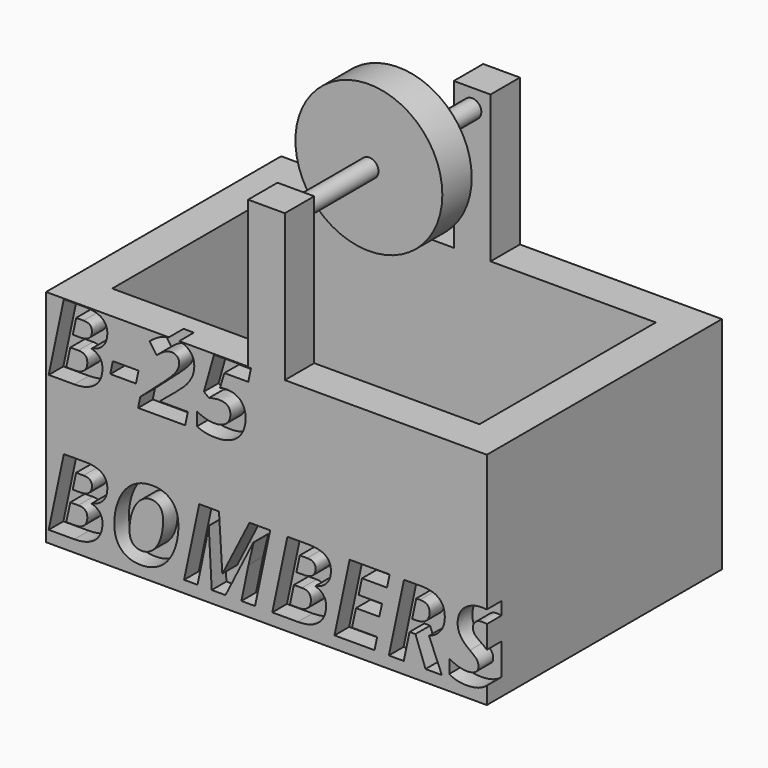
from build123d import *

# Parameters (mm, degrees)
F0_W          = 152.4
F0_H          = 76.2
F1_DEPTH      = 101.6
F2_W          = 127
F2_H          = 76.2
F3_DEPTH      = 63.5
F4_W          = 90.9743383527
F4_H          = 43.2646684349
F5_DEPTH      = 127
F6_W          = 12.7
F6_H          = 12.7
F7_DEPTH      = 50.8
F8_R          = 3.175
F9_DEPTH      = 101.6
F11_R         = 25.4
F12_DEPTH     = 6.35
F15_TEXT_SIZE = 34.6716756447
F16_DEPTH     = 6.35


# Not quite as in the source:
# - the program builds the solid bodies; features that only make, move or delete a surface that nothing else refers to are left out
# - Text() gives the source's letters only with a copy of the font that has no kerning and outlines rounded to 1/6400 em; it was checked with that copy


with BuildPart() as f1:
    # F0 (on Front) → F1 (new body)
    with BuildSketch(Plane.XZ):
        with Locations((-3.6829989403, -13.9763858854)):
            Rectangle(F0_W, F0_H)
    extrude(amount=-F1_DEPTH)

    # F2 (on face) → F3 (cut)
    with BuildSketch(Plane.XY.offset(24.1236141146)):
        with Locations((-3.6829989403, 50.8)):
            Rectangle(F2_W, F2_H)
    extrude(amount=-F3_DEPTH, mode=Mode.SUBTRACT)

    # F4 (on face) → F5 (cut)
    with BuildSketch(Plane.XY.offset(-39.3763858854)):
        with Locations((0.2328343689, 50.1861665398)):
            Rectangle(F4_W, F4_H)
    extrude(amount=-F5_DEPTH, mode=Mode.SUBTRACT)

    # F6 (on face) → F7 (join)
    with BuildSketch(Plane.XY.offset(24.1236141146)):
        with Locations((-3.6829989403, 95.25)):
            Rectangle(F6_W, F6_H)
        with Locations((-3.6829989403, 6.35)):
            Rectangle(F6_W, F6_H)
    extrude(amount=F7_DEPTH)

    # F8 (on face) → F9 (join)
    with BuildSketch(Plane(origin=(0, 101.6, 0), x_dir=(-1, 0, 0), z_dir=(0, 1, 0))):
        with Locations((3.6829989403, 68.5736141146)):
            Circle(F8_R)
    extrude(amount=-F9_DEPTH)

    # F11 (on offset) → F12 (join, symmetric)
    with BuildSketch(Plane.XZ.offset(-50.8)):
        with Locations((-3.8320308086, 68.6379745603)):
            Circle(F11_R)
    extrude(amount=F12_DEPTH, both=True)

    # F15 (on face) → F16 (cut)
    with BuildSketch(Plane.XZ):
        with Locations((-79.8829989403, -0.8399923495)):
            Text('B-25', F15_TEXT_SIZE, font='Open Sans', font_style=FontStyle.BOLDITALIC, text_align=(TextAlign.LEFT, TextAlign.BOTTOM))
        with Locations((-79.8829989403, -47.9934712263)):
            Text('BOMBERS', F15_TEXT_SIZE, font='Open Sans', font_style=FontStyle.BOLDITALIC, text_align=(TextAlign.LEFT, TextAlign.BOTTOM))
    extrude(amount=-F16_DEPTH, mode=Mode.SUBTRACT)


solid = f1.part
